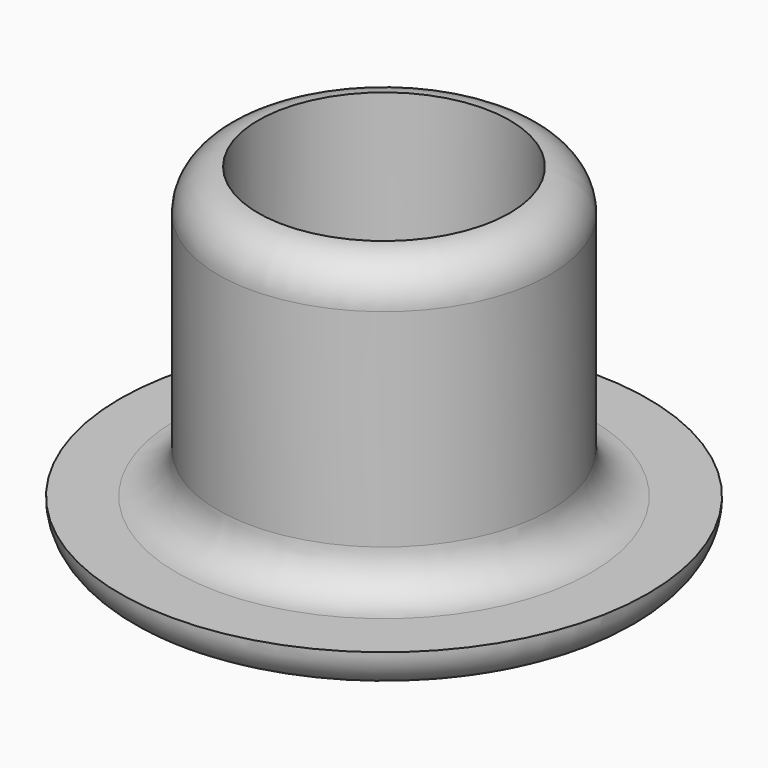
from build123d import *

# Parameters (mm, degrees)
F0_R     = 4
F1_DEPTH = 8
F2_R     = 3.0338863289
F3_DEPTH = 9.4
F4_R     = 6.3699570271
F5_DEPTH = 1
F6_R     = 1


# Not quite as in the source:
# - a fillet or chamfer that OpenCascade refuses, or shapes differently, is made with other operations: its cross-section is extruded or revolved along the edge and cut away or added


with BuildPart() as f1:
    # F0 (on Top) → F1 (new body)
    with BuildSketch(Plane.XY):
        Circle(F0_R)
    extrude(amount=F1_DEPTH)

    # F2 (on Top) → F3 (cut)
    with BuildSketch(Plane.XY):
        Circle(F2_R)
    extrude(amount=F3_DEPTH, mode=Mode.SUBTRACT)

    # F4 (on Top) → F5 (join)
    with BuildSketch(Plane.XY):
        Circle(F4_R)
    extrude(amount=F5_DEPTH)

    # F6
    f6_edges = [f1.edges().sort_by_distance(p)[0] for p in [
        (-4, 0, 1),
    ]]
    fillet(f6_edges, radius=F6_R)

    # F7: fillet of radius 1 on 2 edges, made by hand

    # F7_s1 → F7_t2 (revolve, cut)
    with BuildSketch(Plane.XZ):
        with BuildLine():
            ThreePointArc((6.3699570271, 1), (6.0770638082, 0.2928932188), (5.3699570271, 0))
            Line((5.3699570271, 0), (6.3699570271, 0))
            Line((6.3699570271, 0), (6.3699570271, 1))
        make_face()
    revolve(axis=Axis((0, 0, 0), (0, 0, 1)), mode=Mode.SUBTRACT)

    # F7_s3 → F7_t4 (revolve, cut)
    with BuildSketch(Plane.XZ):
        with BuildLine():
            ThreePointArc((4, 7), (3.7071067812, 7.7071067812), (3, 8))
            Line((3, 8), (4, 8))
            Line((4, 8), (4, 7))
        make_face()
    revolve(axis=Axis((0, 0, 8), (0, 0, 1)), mode=Mode.SUBTRACT)


solid = f1.part
